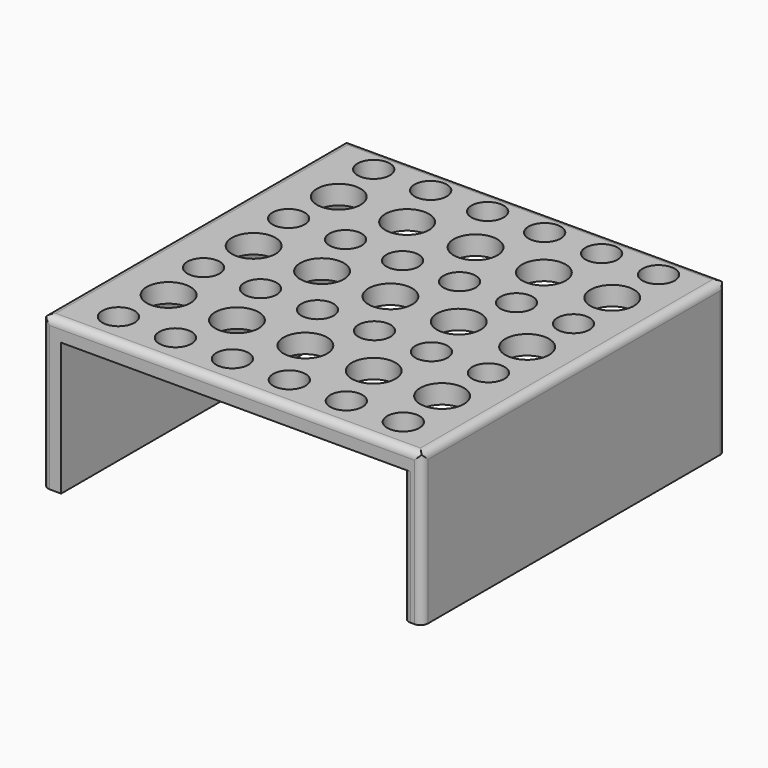
from build123d import *

# Parameters (mm, degrees)
F0_W         = 100
F0_H         = 80
F0_H_2       = 10
F1_DEPTH     = 40
F2_T         = -5
F3_R         = 4.25
F3_R_2       = 5.75
F4_DEPTH     = 40.001
F5_R         = 2
F6_T1_DEPTH  = 48
F6_T3_DEPTH  = 40
F6_T5_DEPTH  = 90
F6_T11_DEPTH = 45
F6_T15_DEPTH = 95
F6_T22_DEPTH = 95
F6_T26_DEPTH = 45
F7_ANGLE     = 180
F8_TEXT_SIZE = 17.3835030066
F9_DEPTH     = 2.5


# Not quite as in the source:
# - a fillet or chamfer that OpenCascade refuses, or shapes differently, is made with other operations: its cross-section is extruded or revolved along the edge and cut away or added
# - Text() gives the source's letters only with a copy of the font that has no kerning and outlines rounded to 1/6400 em; it was checked with that copy


with BuildPart() as f1:
    # F0 (on Top) → F1 (new body)
    with BuildSketch(Plane.XY):
        Rectangle(F0_W, F0_H)
        with Locations((0, 45)):
            Rectangle(F0_W, F0_H_2)
        with Locations((0, -45)):
            Rectangle(F0_W, F0_H_2)
    extrude(amount=F1_DEPTH)

    # F2
    f2_openings = [f1.faces().sort_by_distance(p)[0] for p in [
        (0, 50, 20),
        (0, 0, 40),
        (0, -50, 20),
    ]]
    offset(amount=F2_T, openings=f2_openings)

    # F3 (on face) → F4 (cut, through all)
    with BuildSketch(Plane(origin=(0, 0, 0), x_dir=(1, 0, 0), z_dir=(0, 0, -1))):
        with Locations((7, 13.1419432759)):
            Circle(F3_R)
        with Locations((22, 41.1419432759)):
            Circle(F3_R)
        with Locations((7, -14.8580567241)):
            Circle(F3_R)
        with Locations((17, 27.1419432759)):
            Circle(F3_R_2)
        with Locations((35, -0.8580567241)):
            Circle(F3_R_2)
        with Locations((22, -14.8580567241)):
            Circle(F3_R)
        with Locations((17, -28.8580567241)):
            Circle(F3_R_2)
        with Locations((22, 13.1419432759)):
            Circle(F3_R)
        with Locations((17, -0.8580567241)):
            Circle(F3_R_2)
        with Locations((-1, -0.8580567241)):
            Circle(F3_R_2)
        with Locations((-38, 41.1419432759)):
            Circle(F3_R)
        with Locations((7, 41.1419432759)):
            Circle(F3_R)
        with Locations((37, -14.8580567241)):
            Circle(F3_R)
        with Locations((-23, 13.1419432759)):
            Circle(F3_R)
        with Locations((35, 27.1419432759)):
            Circle(F3_R_2)
        with Locations((37, 13.1419432759)):
            Circle(F3_R)
        with Locations((-23, 41.1419432759)):
            Circle(F3_R)
        with Locations((-8, -14.8580567241)):
            Circle(F3_R)
        with Locations((-8, 13.1419432759)):
            Circle(F3_R)
        with Locations((-8, 41.1419432759)):
            Circle(F3_R)
        with Locations((7, -42.8580567241)):
            Circle(F3_R)
        with Locations((37, -42.8580567241)):
            Circle(F3_R)
        with Locations((35, -28.8580567241)):
            Circle(F3_R_2)
        with Locations((-19, 27.1419432759)):
            Circle(F3_R_2)
        with Locations((22, -42.8580567241)):
            Circle(F3_R)
        with Locations((-1, 27.1419432759)):
            Circle(F3_R_2)
        with Locations((37, 41.1419432759)):
            Circle(F3_R)
        with Locations((-1, -28.8580567241)):
            Circle(F3_R_2)
        with Locations((-38, -14.8580567241)):
            Circle(F3_R)
        with Locations((-38, 13.1419432759)):
            Circle(F3_R)
        with Locations((-19, -0.8580567241)):
            Circle(F3_R_2)
        with Locations((-37, -0.8580567241)):
            Circle(F3_R_2)
        with Locations((-23, -42.8580567241)):
            Circle(F3_R)
        with Locations((-23, -14.8580567241)):
            Circle(F3_R)
        with Locations((-8, -42.8580567241)):
            Circle(F3_R)
        with Locations((-37, 27.1419432759)):
            Circle(F3_R_2)
        with Locations((-19, -28.8580567241)):
            Circle(F3_R_2)
        with Locations((-37, -28.8580567241)):
            Circle(F3_R_2)
        with Locations((-38, -42.8580567241)):
            Circle(F3_R)
    extrude(amount=-F4_DEPTH, mode=Mode.SUBTRACT)

    # F5
    f5_edges = [f1.edges().sort_by_distance(p)[0] for p in [
        (0, 50, 0),
        (-50, 0, 0),
        (0, -50, 0),
        (50, 0, 0),
    ]]
    fillet(f5_edges, radius=F5_R)

    # F6: fillet of radius 2 on 11 edges, made by hand

    # F6_s2 → F6_t1 (cut)
    with BuildSketch(Plane.XY.offset(-3)):
        with BuildLine():
            ThreePointArc((-50, 48), (-49.4142135624, 49.4142135624), (-48, 50))
            Line((-48, 50), (-50, 50))
            Line((-50, 50), (-50, 48))
        make_face()
        with BuildLine():
            ThreePointArc((48, 50), (49.4142135624, 49.4142135624), (50, 48))
            Line((50, 48), (50, 50))
            Line((50, 50), (48, 50))
        make_face()
        with BuildLine():
            ThreePointArc((48, -50), (49.4142135624, -49.4142135624), (50, -48))
            Line((50, -48), (50, -50))
            Line((50, -50), (48, -50))
        make_face()
        with BuildLine():
            ThreePointArc((-50, -48), (-49.4142135624, -49.4142135624), (-48, -50))
            Line((-48, -50), (-50, -50))
            Line((-50, -50), (-50, -48))
        make_face()
    extrude(amount=F6_T1_DEPTH, mode=Mode.SUBTRACT)

    # F6_s4 → F6_t3 (cut)
    with BuildSketch(Plane.XY.offset(5)):
        with BuildLine():
            ThreePointArc((-47, 50), (-45.5857864376, 49.4142135624), (-45, 48))
            Line((-45, 48), (-45, 50))
            Line((-45, 50), (-47, 50))
        make_face()
        with BuildLine():
            ThreePointArc((47, 50), (45.5857864376, 49.4142135624), (45, 48))
            Line((45, 48), (45, 50))
            Line((45, 50), (47, 50))
        make_face()
        with BuildLine():
            ThreePointArc((-47, -50), (-45.5857864376, -49.4142135624), (-45, -48))
            Line((-45, -48), (-45, -50))
            Line((-45, -50), (-47, -50))
        make_face()
    extrude(amount=F6_T3_DEPTH, mode=Mode.SUBTRACT)

    # F6_s6 → F6_t5 (cut)
    with BuildSketch(Plane.YZ.offset(-45)):
        with BuildLine():
            ThreePointArc((50, 3), (49.4142135624, 4.4142135624), (48, 5))
            Line((48, 5), (50, 5))
            Line((50, 5), (50, 3))
        make_face()
    extrude(amount=F6_T5_DEPTH, mode=Mode.SUBTRACT)


with BuildPart() as f6_tool9:
    # F6_s10 → F6_t11 (new body)
    with BuildSketch(Plane.XY):
        with BuildLine():
            ThreePointArc((-47, 50), (-45.5857864376, 49.4142135624), (-45, 48))
            Line((-45, 48), (-45, 50))
            Line((-45, 50), (-47, 50))
        make_face()
    extrude(amount=F6_T11_DEPTH)

    split(bisect_by=Plane.XY.offset(5), keep=Keep.BOTTOM)


with BuildPart() as f6_tool13:
    # F6_s14 → F6_t15 (new body)
    with BuildSketch(Plane.YZ.offset(45)):
        with BuildLine():
            ThreePointArc((50, 3), (49.4142135624, 4.4142135624), (48, 5))
            Line((48, 5), (50, 5))
            Line((50, 5), (50, 3))
        make_face()
    extrude(amount=-F6_T15_DEPTH)

    split(bisect_by=Plane.YZ.offset(-45), keep=Keep.BOTTOM)


with BuildPart() as f6_tool9_1:
    add(f6_tool9.part)

    # F6_t17: intersect F6_tool13
    add(f6_tool13.part, mode=Mode.INTERSECT)


with BuildPart() as f1_1:
    add(f1.part)

    # F6_t7: cut F6_tool9
    add(f6_tool9_1.part, mode=Mode.SUBTRACT)


with BuildPart() as f6_tool20:
    # F6_s21 → F6_t22 (new body)
    with BuildSketch(Plane.YZ.offset(50)):
        with BuildLine():
            ThreePointArc((50, 3), (49.4142135624, 4.4142135624), (48, 5))
            Line((48, 5), (50, 5))
            Line((50, 5), (50, 3))
        make_face()
    extrude(amount=-F6_T22_DEPTH)

    split(bisect_by=Plane.YZ.offset(45), keep=Keep.TOP)


with BuildPart() as f6_tool24:
    # F6_s25 → F6_t26 (new body)
    with BuildSketch(Plane.XY):
        with BuildLine():
            ThreePointArc((47, 50), (45.5857864376, 49.4142135624), (45, 48))
            Line((45, 48), (45, 50))
            Line((45, 50), (47, 50))
        make_face()
    extrude(amount=F6_T26_DEPTH)

    split(bisect_by=Plane.XY.offset(5), keep=Keep.BOTTOM)


with BuildPart() as f6_tool20_1:
    add(f6_tool20.part)

    # F6_t28: intersect F6_tool24
    add(f6_tool24.part, mode=Mode.INTERSECT)


with BuildPart() as f1_2:
    add(f1_1.part)

    # F6_t18: cut F6_tool20
    add(f6_tool20_1.part, mode=Mode.SUBTRACT)


with BuildPart() as f1_3:
    # F7: moved
    add(f1_2.part.rotate(Axis((-45, 0, 5), (0, -1, 0)), F7_ANGLE))

    # F8 (on face) → F9 (cut)
    with BuildSketch(Plane(origin=(-140, 0, 0), x_dir=(0, -1, 0), z_dir=(-1, 0, 0))):
        with Locations((16.0758834779, -26.9043321908)):
            Text('D H', F8_TEXT_SIZE, font='Open Sans', text_align=(TextAlign.LEFT, TextAlign.BOTTOM))
    extrude(amount=-F9_DEPTH, mode=Mode.SUBTRACT)


solid = f1_3.part
